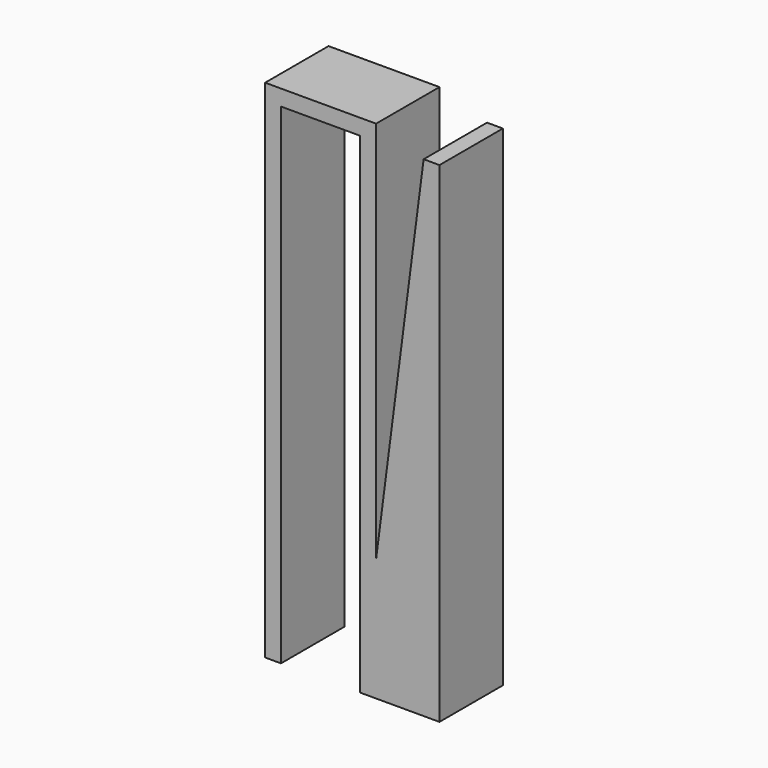
from build123d import *

# Parameters (mm, degrees)
F1_DEPTH   = 25
F1_FACE_W  = 5
F1_FACE_H  = 25
F1_FACE1_W = 25
F1_FACE1_H = 25


with BuildPart() as f1:
    # F0 (on Front) → F1 (new body)
    with BuildSketch(Plane.XZ):
        Polygon((0, -93.0193822413), (0, 61.6336810916), (25, 61.6336810916), (25, -93.0193822413), (50, -93.0193822413), (50, 61.6336810916), (45, 61.6336810916), (45, -88.0193822413), (30, -88.0193822413), (30, 66.6336810916), (-5, 66.6336810916), (-5, -93.0193822413), align=None)
    extrude(amount=F1_DEPTH)

    # F1_face (on face) → F2 section 0
    with BuildSketch(Plane(origin=(47.5, -12.5, 61.6336810916), x_dir=(1, 0, 0), z_dir=(0, 0, 1))):
        Rectangle(F1_FACE_W, F1_FACE_H)
    # F1_face1 (on face) → F2 section 1
    with BuildSketch(Plane(origin=(37.5, -12.5, -93.0193822413), x_dir=(1, 0, 0), z_dir=(0, 0, -1))):
        Rectangle(F1_FACE1_W, F1_FACE1_H)
    loft()


solid = f1.part
